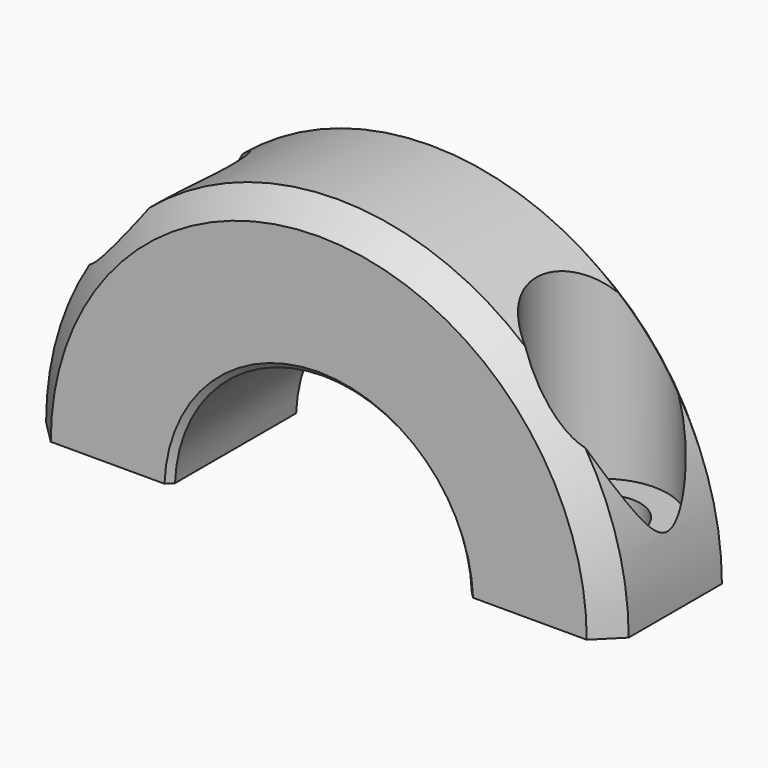
from build123d import *

# Parameters (mm, degrees)
F1_DEPTH       = 14
F4_D           = 6.6
F4_DEPTH       = 30
F4_CBORE_D     = 11.25
F4_CBORE_DEPTH = 20
F4_TIP         = 1.9828400428
F5_T2_ANGLE    = 203.6133668192
F5_T4_ANGLE    = 203.6133668192
F6_SIZE        = 0.5


# Not quite as in the source:
# - a fillet or chamfer that OpenCascade refuses, or shapes differently, is made with other operations: its cross-section is extruded or revolved along the edge and cut away or added


with BuildPart() as f1:
    # F0 (on Front) → F1 (new body)
    with BuildSketch(Plane.XZ):
        with BuildLine():
            Line((12.7401923062, 0), (25, 0))
            ThreePointArc((25, 0), (0, 25), (-25, 0))
            Line((-25, 0), (-12.7401923062, 0))
            ThreePointArc((-12.7401923062, 0), (0, 12.25), (12.7401923062, 0))
        make_face()
    extrude(amount=F1_DEPTH)

    # F4
    with Locations(Plane.XY.offset(25)):
        with Locations((-18.7, -7), (18.7, -7)):
            CounterBoreHole(F4_D / 2, F4_CBORE_D / 2, F4_CBORE_DEPTH, depth=F4_DEPTH)
            with Locations((0, 0, -(F4_DEPTH + F4_TIP / 2))):  # 118° drill point
                Cone(0, F4_D / 2, F4_TIP, mode=Mode.SUBTRACT)

    # F5: chamfer of 2 on 2 edges, made by hand

    # F5_s1 → F5_t2 (revolve, cut)
    with BuildSketch(Plane(origin=(0, 0, 0), x_dir=(0, 1, 0), z_dir=(-0.2046102329, 0, -0.9788435281))):
        Polygon((-12, 25), (-14, 23), (-14, 25), align=None)
    revolve(axis=Axis((0, -14, 0), (0, -1, 0)), revolution_arc=F5_T2_ANGLE, mode=Mode.SUBTRACT)

    # F5_s3 → F5_t4 (revolve, cut)
    with BuildSketch(Plane(origin=(0, 0, 0), x_dir=(0, 1, 0), z_dir=(-0.2046102329, 0, -0.9788435281))):
        Polygon((-2, 25), (0, 23), (0, 25), align=None)
    revolve(axis=Axis((0, 0, 0), (0, -1, 0)), revolution_arc=F5_T4_ANGLE, mode=Mode.SUBTRACT)

    # F6
    f6_edges = [f1.edges().sort_by_distance(p)[0] for p in [
        (0, -14, 12.25),
        (0, 0, 12.25),
    ]]
    chamfer(f6_edges, length=F6_SIZE)


solid = f1.part
